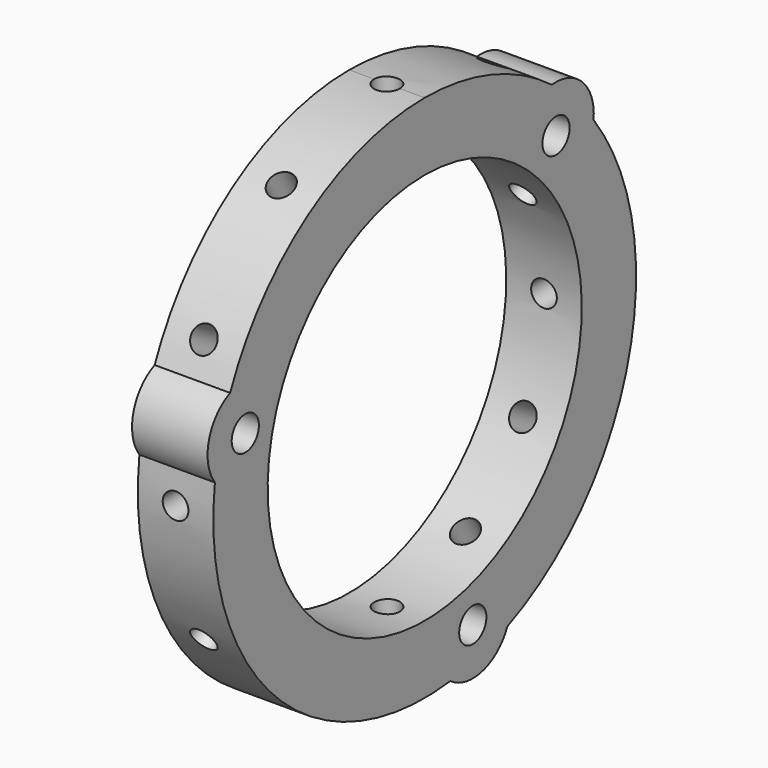
from build123d import *

# Parameters (mm, degrees)
F0_W            = 20
F0_H            = 18
F2_R            = 3.4
F3_DEPTH        = 100
F3_COPIES_COUNT = 12
F4_R            = 4.5
F5_DEPTH        = 20
F5_COPIES_COUNT = 3
F7_DEPTH        = 20


# Not quite as in the source:
# - a pattern or mirror of a feature is missing from the dataset's text; its kind, count and spacing are read off the source's solid


with BuildPart() as f1:
    # F0 (on Front) → F1 (revolve)
    with BuildSketch(Plane.XZ):
        with Locations((-10, 61)):
            Rectangle(F0_W, F0_H)
    revolve(axis=Axis((-48.3428524689, 0, 0), (-1, 0, 0)))

    # F2 (on Top) → F3 (cut)
    with BuildSketch(Plane.XY):
        with Locations((-10, 0)):
            Circle(F2_R)
    f3 = extrude(amount=F3_DEPTH, mode=Mode.SUBTRACT)

    # F3_copies: F3 ×12 about axis
    f3_copies_axis = Axis((0, 0, 0), (1, 0, 0))
    for i in range(1, F3_COPIES_COUNT):
        add(f3.rotate(f3_copies_axis, i * 360 / F3_COPIES_COUNT), mode=Mode.SUBTRACT)

    # F4 (on Right) → F5 (cut, symmetric)
    with BuildSketch(Plane.YZ):
        with Locations((43.487067043, 43.487067043)):
            Circle(F4_R)
    f5 = extrude(amount=F5_DEPTH, both=True, mode=Mode.SUBTRACT)

    # F5_copies: F5 ×3 about axis
    f5_copies_axis = Axis((0, 0, 0), (1, 0, 0))
    for i in range(1, F5_COPIES_COUNT):
        add(f5.rotate(f5_copies_axis, i * 360 / F5_COPIES_COUNT), mode=Mode.SUBTRACT)

    # F6 (on Right) → F7 (join)
    with BuildSketch(Plane.YZ):
        with BuildLine():
            ThreePointArc((-69.4797099698, 8.5187970112), (-67.6148078402, 18.1173331572), (-64.430592387, 27.3623603635))
            ThreePointArc((-64.430592387, 27.3623603635), (-71.4785111454, 19.1526093376), (-69.4797099698, 8.5187970112))
        make_face()
        with BuildLine():
            ThreePointArc((27.3623603635, -64.430592387), (18.1173331572, -67.6148078402), (8.5187970112, -69.4797099698))
            ThreePointArc((8.5187970112, -69.4797099698), (19.1526093376, -71.4785111454), (27.3623603635, -64.430592387))
        make_face()
        with BuildLine():
            ThreePointArc((42.1173496063, 55.9117953758), (49.4974746831, 49.4974746831), (55.9117953758, 42.1173496063))
            ThreePointArc((55.9117953758, 42.1173496063), (52.3259018078, 52.3259018078), (42.1173496063, 55.9117953758))
        make_face()
    extrude(amount=-F7_DEPTH)


solid = f1.part
